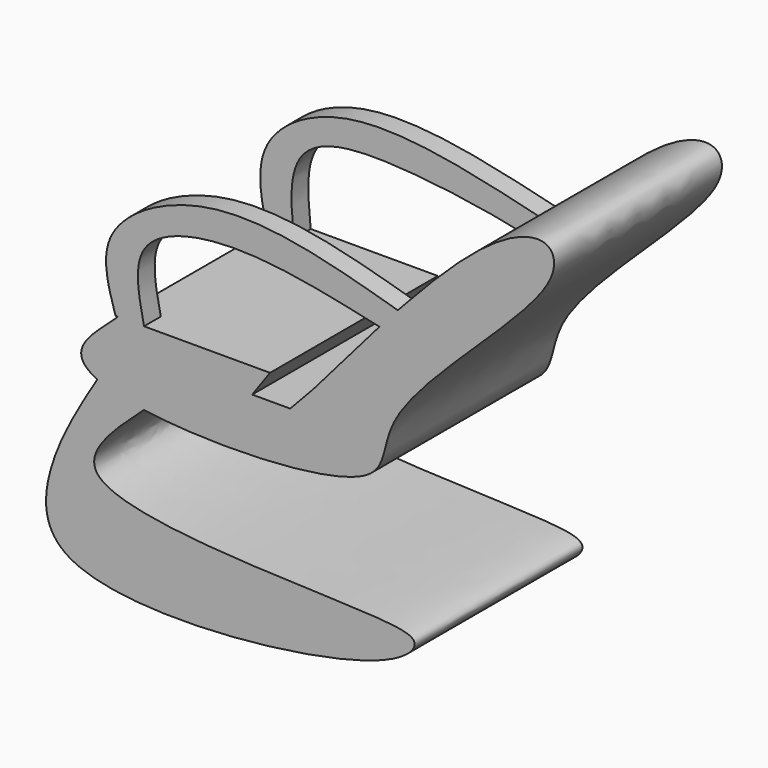
from build123d import *

# Parameters (mm, degrees)
F1_DEPTH = 50.8
F3_DEPTH = 50.8
F5_DEPTH = 5.08
F8_DEPTH = 5.08


with BuildPart() as f1:
    # F0 (on Front) → F1 (new body)
    with BuildSketch(Plane.XZ):
        with BuildLine():
            add(Edge.make_bspline(
                [(1.3720039788, 24.2892022985), (1.7397140704, 24.3971631629), (1.7582926908, 24.568888641), (1.7823616223, 24.7359291989)],
                knots=[0.9509189129, 0.9509189129, 0.9509189129, 0.9509189129, 1, 1, 1, 1], degree=3))
            add(Edge.make_bspline(
                [(1.3720039788, 24.2892022985), (1.5089424114, 24.4385087599), (1.645729306, 24.5874203671), (1.7823616223, 24.7359291989)],
                knots=[0.0847794827, 0.0847794827, 0.0847794827, 0.0847794827, 0.0864803054, 0.0864803054, 0.0864803054, 0.0864803054], degree=3))
        make_face()
        with BuildLine():
            add(Edge.make_bspline(
                [(1.7823616223, 24.7359291989), (10.4049223213, 34.1079902909), (24.6949847785, 47.9715643142), (38.1344093391, 51.2484791452), (40.2493490628, 37.4143547222), (-6.5236955819, 2.184894081), (0.9253594538, -18.8463747396), (-43.6446723435, -20.3182131852), (-60.9473315781, -17.832391591)],
                knots=[0.0864803054, 0.0864803054, 0.0864803054, 0.0864803054, 0.1938154316, 0.2780423559, 0.3466486519, 0.5259158447, 0.6216858734, 0.7851855678, 0.7851855678, 0.7851855678, 0.7851855678], degree=3))
            add(Edge.make_bspline(
                [(1.3720039788, 24.2892022985), (1.7397140704, 24.3971631629), (1.7582926908, 24.568888641), (1.7823616223, 24.7359291989)],
                knots=[0.9509189129, 0.9509189129, 0.9509189129, 0.9509189129, 1, 1, 1, 1], degree=3))
            add(Edge.make_bspline(
                [(-19.8585968465, 0), (-12.6562240513, 8.4234241533), (-5.4538512561, 16.8468483066), (1.3720039788, 24.2892022985)],
                knots=[0, 0, 0, 0, 0.0847794827, 0.0847794827, 0.0847794827, 0.0847794827], degree=3))
            Line((-19.8585968465, 0), (-59.575792402, 0))
            Line((-59.575792402, 0), (-67.3465505242, 0))
            add(Edge.make_bspline(
                [(-72.2228055042, -15.0039612217), (-75.6102264743, -13.4364498149), (-78.647523508, -8.5551664347), (-67.4293044875, -0.7769035344), (-67.3465505242, 0)],
                knots=[0.8303948244, 0.8303948244, 0.8303948244, 0.8303948244, 0.8895952068, 0.9740693054, 0.9740693054, 0.9740693054, 0.9740693054], degree=3))
            add(Edge.make_bspline(
                [(-60.9473315781, -17.832391591), (-63.6766425714, -17.4402795975), (-67.9897670224, -16.6040196588), (-71.1116634352, -15.5181364254), (-72.2228055042, -15.0039612217)],
                knots=[0.7851855678, 0.7851855678, 0.7851855678, 0.7851855678, 0.8109759107, 0.8303948244, 0.8303948244, 0.8303948244, 0.8303948244], degree=3))
        make_face()
        with BuildLine():
            add(Edge.make_bspline(
                [(-60.9473315781, -17.832391591), (-68.3398865258, -24.5026777809), (-89.1217537647, -43.2708973163), (-5.3227975989, -42.4290767481), (7.4812685723, -45.5794694888), (-5.8275820787, -57.5943863726), (-86.1957011785, -65.2412145747), (-85.0369884931, -36.1539051668), (-76.7094239518, -22.4026879312), (-72.2228055042, -15.0039612217)],
                knots=[0, 0, 0, 0, 0.1222593736, 0.3434667497, 0.4265239574, 0.5203698368, 0.750455011, 0.8648549189, 1, 1, 1, 1], degree=3))
            add(Edge.make_bspline(
                [(-60.9473315781, -17.832391591), (-63.6766425714, -17.4402795975), (-67.9897670224, -16.6040196588), (-71.1116634352, -15.5181364254), (-72.2228055042, -15.0039612217)],
                knots=[0.7851855678, 0.7851855678, 0.7851855678, 0.7851855678, 0.8109759107, 0.8303948244, 0.8303948244, 0.8303948244, 0.8303948244], degree=3))
        make_face()
    extrude(amount=F1_DEPTH)

    # F2 (on face) → F3 (cut)
    with BuildSketch(Plane.XZ.offset(50.8)):
        Polygon((-25.5126804113, -6.0439207591), (-19.8585968465, 0), (-30.4053779691, 0), (-34.7224660218, -6.0439207591), align=None)
    extrude(amount=-F3_DEPTH, mode=Mode.SUBTRACT)

    # F4 (on Front) → F5 (join)
    with BuildSketch(Plane.XZ):
        with BuildLine():
            Line((-67.8186118603, 0), (-61.199080199, 0))
            add(Edge.make_bspline(
                [(-61.199080199, 0), (-61.7739967068, 5.7786274101), (-62.9465941346, 17.5646929419), (-47.7710562815, 27.5388880245), (-1.8008547484, 19.0708813453), (-2.8174213014, 17.8499860268), (-2.7888165903, 17.6540961534), (-2.7745142579, 17.5561513752)],
                knots=[0, 0, 0, 0, 0.2527959656, 0.5156016482, 0.931848526, 0.9659243181, 1, 1, 1, 1], degree=3))
            Line((-2.7745142579, 17.5561513752), (0, 23.6000716686))
            add(Edge.make_bspline(
                [(-67.8186118603, 0), (-69.084130238, 5.9195330657), (-71.8246062407, 18.7382630022), (-47.3330869592, 35.1157333271), (-17.6301382902, 27.8893061256), (0, 23.6000716686)],
                knots=[0, 0, 0, 0, 0.258565474, 0.5599227076, 1, 1, 1, 1], degree=3))
        make_face()
    extrude(amount=F5_DEPTH)

    # F7 (on offset) → F8 (join)
    with BuildSketch(Plane.XZ.offset(50.8)):
        with BuildLine():
            add(Edge.make_bspline(
                [(-67.8186118603, 0), (-69.5651200636, 5.6305472506), (-73.5767857211, 18.5637089699), (-43.3104422795, 36.086276428), (-15.0319972981, 27.9071176477), (0.9593538707, 23.2818350196)],
                knots=[0, 0, 0, 0, 0.2509454521, 0.5764125528, 1, 1, 1, 1], degree=3))
            Line((-67.8186118603, 0), (-60.9112754464, 0))
            add(Edge.make_bspline(
                [(-60.9112754464, 0), (-62.1938366242, 6.0913837059), (-64.9104445252, 18.9936151087), (-39.7479924583, 26.4162692115), (-16.5673294946, 21.2527126033), (-3.1154335011, 18.2562656701)],
                knots=[0, 0, 0, 0, 0.2729170634, 0.5780688388, 1, 1, 1, 1], degree=3))
            Line((-3.1154335011, 18.2562656701), (0.9593538707, 23.2818350196))
        make_face()
    extrude(amount=-F8_DEPTH)


solid = f1.part
